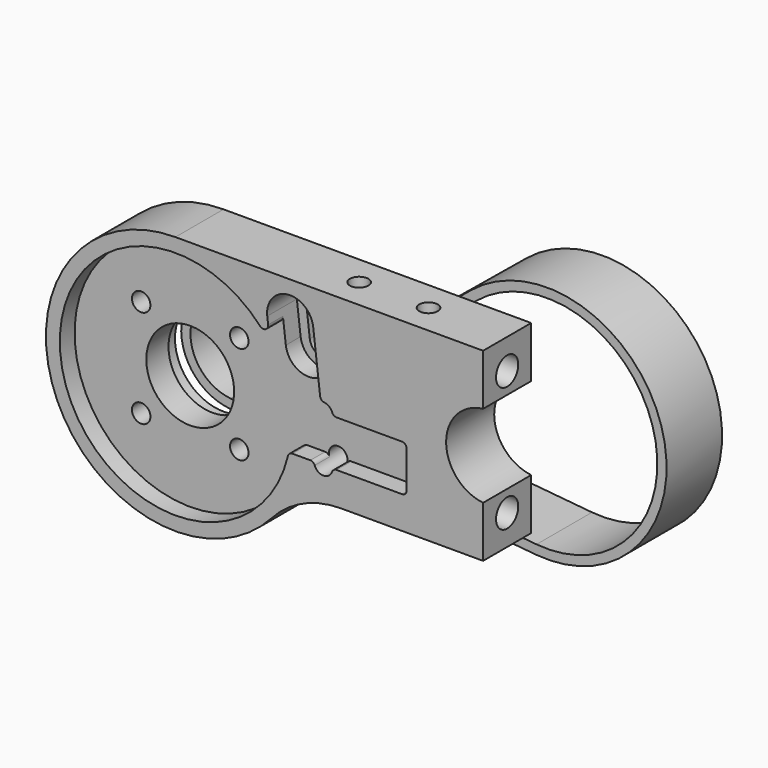
from build123d import *

# Parameters (mm, degrees)
F0_R         = 2
F0_R_2       = 9
F1_DEPTH     = 9
F2_R         = 9.5
F3_DEPTH     = 9
F4_R         = 25
F5_DEPTH     = 4
F8_DEPTH     = 8
F10_DEPTH    = 5.001
F11_R        = 1
F13_DEPTH    = 4
F14_R        = 1
F16_R        = 2
F17_DEPTH    = 13.001
F18_T1_DEPTH = 6.0710678119
F18_T3_DEPTH = 6.4150512427
F20_DEPTH    = 3
F21_R        = 3
F22_DEPTH    = 14
F25_DEPTH    = 15
F26_R        = 2
F27_DEPTH    = 14
F28_R        = 3.75
F29_DEPTH    = 3.5
F30_R        = 10.5
F31_DEPTH    = 3


# Not quite as in the source:
# - a fillet or chamfer that OpenCascade refuses, or shapes differently, is made with other operations: its cross-section is extruded or revolved along the edge and cut away or added


with BuildPart() as f1:
    # F0 (on Front) → F1 (new body)
    with BuildSketch(Plane.XZ):
        with BuildLine():
            ThreePointArc((66.5277720645, -0.94427191), (58.5277720645, 8), (66.5277720645, 16.94427191))
            Line((66.5277720645, 16.94427191), (66.5277720645, 28))
            Line((66.5277720645, 28), (0, 28))
            ThreePointArc((0, 28), (-25.5603860169, -11.430952133), (20.86996779, -18.6666666667))
            ThreePointArc((20.86996779, -18.6666666667), (27.6121218307, -13.7425814165), (35.77708764, -12))
            Line((35.77708764, -12), (66.5277720645, -12))
            Line((66.5277720645, -12), (66.5277720645, -0.94427191))
        make_face()
        with Locations((-10.6066017178, -10.6066017178)):
            Circle(F0_R, mode=Mode.SUBTRACT)
        with Locations((10.6066017178, -10.6066017178)):
            Circle(F0_R, mode=Mode.SUBTRACT)
        with Locations((-10.6066017178, 10.6066017178)):
            Circle(F0_R, mode=Mode.SUBTRACT)
        Circle(F0_R_2, mode=Mode.SUBTRACT)
        with Locations((10.6066017178, 10.6066017178)):
            Circle(F0_R, mode=Mode.SUBTRACT)
    extrude(amount=F1_DEPTH)

    # F2 (on face) → F3 (cut)
    with BuildSketch(Plane(origin=(0, 0, 0), x_dir=(-1, 0, 0), z_dir=(0, 1, 0))):
        Circle(F2_R)
    extrude(amount=-F3_DEPTH, mode=Mode.SUBTRACT)

    # F4 (on face) → F5 (join)
    with BuildSketch(Plane.XZ.offset(9)):
        with BuildLine():
            Line((66.5277720645, 28), (0, 28))
            ThreePointArc((0, 28), (-25.5603860169, -11.430952133), (20.86996779, -18.6666666667))
            ThreePointArc((20.86996779, -18.6666666667), (27.6121218307, -13.7425814165), (35.77708764, -12))
            Line((35.77708764, -12), (66.5277720645, -12))
            Line((66.5277720645, -12), (66.5277720645, -0.94427191))
            ThreePointArc((66.5277720645, -0.94427191), (58.5277720645, 8), (66.5277720645, 16.94427191))
            Line((66.5277720645, 16.94427191), (66.5277720645, 28))
        make_face()
        Circle(F4_R, mode=Mode.SUBTRACT)
    extrude(amount=F5_DEPTH)

    # F7 (on face) → F8 (cut)
    with BuildSketch(Plane.XZ.offset(13)):
        with BuildLine():
            ThreePointArc((20.6707497856, 12.5187900095), (26.2242624374, 8.1417479459), (30.601304501, 13.6952605977))
            Line((30.601304501, 13.6952605977), (29.7846953358, 20.5882352941))
            ThreePointArc((29.7846953358, 20.5882352941), (24.231182684, 24.9652773577), (19.8541406204, 19.4117647059))
            Line((19.8541406204, 19.4117647059), (20.6707497856, 12.5187900095))
        make_face()
    extrude(amount=-F8_DEPTH, mode=Mode.SUBTRACT)

    # F9 (on face) → F10 (cut, through all)
    with BuildSketch(Plane.XZ.offset(5)):
        with BuildLine():
            ThreePointArc((27.7985843927, 20.3529411765), (24.4664768016, 22.9791664146), (21.8402515635, 19.6470588235))
            Line((21.8402515635, 19.6470588235), (22.6568607287, 12.7540841271))
            ThreePointArc((22.6568607287, 12.7540841271), (25.9889683197, 10.127858889), (28.6151935579, 13.4599664801))
            Line((28.6151935579, 13.4599664801), (27.7985843927, 20.3529411765))
        make_face()
    extrude(amount=-F10_DEPTH, mode=Mode.SUBTRACT)

    # F11
    f11_edges = [f1.edges().sort_by_distance(p)[0] for p in [
        (20.450239, -11, 14.380116),
        (23.474902, -11, 8.598196),
    ]]
    fillet(f11_edges, radius=F11_R)

    # F12 (on face) → F13 (cut, through all)
    with BuildSketch(Plane.XZ.offset(13)):
        with BuildLine():
            ThreePointArc((24.038630661, 6.8661660296), (24.9815394091, 0.9605668915), (24.4948974278, -5))
            Line((24.4948974278, -5), (50, -5))
            Line((50, -5), (50, 0))
            Line((50, 0), (50, 5))
            Line((50, 5), (31.6314300723, 5))
            Line((31.6314300723, 5), (30.601304501, 13.6952605977))
            ThreePointArc((30.601304501, 13.6952605977), (29.192263391, 9.5923156783), (25.1061510967, 8.1351814429))
            ThreePointArc((25.1061510967, 8.1351814429), (24.2349308003, 7.7845517146), (24.038630661, 6.8661660296))
        make_face()
    extrude(amount=-F13_DEPTH, mode=Mode.SUBTRACT)

    # F14
    f14_edges = [f1.edges().sort_by_distance(p)[0] for p in [
        (24.494897, -11, -5),
        (50, -11, 5),
        (50, -11, -5),
    ]]
    fillet(f14_edges, radius=F14_R)

    # F16 (on face) → F17 (cut, through all)
    with BuildSketch(Plane.XZ.offset(13)):
        with Locations((32, 5)):
            Circle(F16_R)
        with Locations((32, -5)):
            Circle(F16_R)
    extrude(amount=-F17_DEPTH, mode=Mode.SUBTRACT)

    # F18: fillet of radius 1 on 4 edges, made by hand

    # F18_s2 → F18_t1 (cut)
    with BuildSketch(Plane.XZ.offset(9)):
        with BuildLine():
            ThreePointArc((34.8284271248, -5), (34.2510768556, -5.1835034191), (33.8856180832, -5.6666666667))
            ThreePointArc((33.8856180832, -5.6666666667), (33.9711971193, -5.3382039575), (34, -5))
            Line((34, -5), (34.8284271248, -5))
        make_face()
        with BuildLine():
            ThreePointArc((29.1715728752, -5), (29.7489231444, -5.1835034191), (30.1143819168, -5.6666666667))
            ThreePointArc((30.1143819168, -5.6666666667), (30.0288028807, -5.3382039575), (30, -5))
            Line((30, -5), (29.1715728752, -5))
        make_face()
        with BuildLine():
            ThreePointArc((34.8284271248, 5), (34.2510768556, 5.1835034191), (33.8856180832, 5.6666666667))
            ThreePointArc((33.8856180832, 5.6666666667), (33.9711971193, 5.3382039575), (34, 5))
            Line((34, 5), (34.8284271248, 5))
        make_face()
    extrude(amount=F18_T1_DEPTH, mode=Mode.SUBTRACT)

    # F18_s4 → F18_t3 (cut)
    with BuildSketch(Plane.XZ.offset(9)):
        with BuildLine():
            ThreePointArc((32.1897446196, 6.9909788998), (31.5856544625, 7.2713099967), (31.2915614579, 7.8688212908))
            Line((31.2915614579, 7.8688212908), (31.4052109282, 6.9095093506))
            ThreePointArc((31.4052109282, 6.9095093506), (31.7934217487, 6.9893027487), (32.1897446196, 6.9909788998))
        make_face()
    extrude(amount=F18_T3_DEPTH, mode=Mode.SUBTRACT)

    # F19 (on face) → F20 (cut)
    with BuildSketch(Plane(origin=(0, 0, 0), x_dir=(-1, 0, 0), z_dir=(0, 1, 0))):
        with BuildLine():
            ThreePointArc((-30, 5), (-32, 7), (-34, 5))
            Line((-34, 5), (-34, -5))
            ThreePointArc((-34, -5), (-32, -7), (-30, -5))
            Line((-30, -5), (-30, 5))
        make_face()
    extrude(amount=-F20_DEPTH, mode=Mode.SUBTRACT)

    # F21 (on face) → F22 (cut)
    with BuildSketch(Plane.YZ.offset(66.5277720645)):
        with Locations((-6.5, 21.5)):
            Circle(F21_R)
        with Locations((-6.5, -5.5)):
            Circle(F21_R)
    extrude(amount=-F22_DEPTH, mode=Mode.SUBTRACT)

    # F26 (on face) → F27 (cut)
    with BuildSketch(Plane.XY.offset(28)):
        with Locations((49.5277720645, -6.5)):
            Circle(F26_R)
        with Locations((34.5277720645, -6.5)):
            Circle(F26_R)
    extrude(amount=-F27_DEPTH, mode=Mode.SUBTRACT)

    # F28 (on face) → F29 (cut)
    with BuildSketch(Plane(origin=(0, 0, 0), x_dir=(-1, 0, 0), z_dir=(0, 1, 0))):
        with Locations((-10.6066017178, -10.6066017178)):
            Circle(F28_R)
        with Locations((10.6066017178, -10.6066017178)):
            Circle(F28_R)
        with Locations((10.6066017178, 10.6066017178)):
            Circle(F28_R)
        with Locations((-10.6066017178, 10.6066017178)):
            Circle(F28_R)
    extrude(amount=-F29_DEPTH, mode=Mode.SUBTRACT)

    # F30 (on face) → F31 (cut)
    with BuildSketch(Plane(origin=(0, 0, 0), x_dir=(-1, 0, 0), z_dir=(0, 1, 0))):
        Circle(F30_R)
    extrude(amount=-F31_DEPTH, mode=Mode.SUBTRACT)


with BuildPart() as f25:
    # F24 (on offset) → F25 (new body)
    with BuildSketch(Plane(origin=(0, 3, 0), x_dir=(-1, 0, 0), z_dir=(0, 1, 0))):
        with BuildLine():
            Line((-30.2365222754, 10.8918314545), (-51.1259867982, 28.0124227688))
            ThreePointArc((-51.1259867982, 28.0124227688), (-92.2766057305, 15.5505534348), (-65.0905572844, -17.759961357))
            Line((-65.0905572844, -17.759961357), (1.0879161627, -11.4986494173))
            ThreePointArc((1.0879161627, -11.4986494173), (11.4944642154, 1.1312790991), (-1.1746259412, 11.4901154867))
            Line((-1.1746259412, 11.4901154867), (-24.3518451825, 9.1207256405))
            ThreePointArc((-24.3518451825, 9.1207256405), (-27.471031774, 9.4186831416), (-30.2365222754, 10.8918314545))
        make_face()
        with BuildLine():
            ThreePointArc((-65.2789410355, -15.7688532328), (-90.3636524037, 14.966935778), (-52.39375764, 26.4655688349))
            Line((-52.39375764, 26.4655688349), (-31.5042931172, 9.3449775207))
            ThreePointArc((-31.5042931172, 9.3449775207), (-28.0474299905, 7.5035421295), (-24.1484467511, 7.1310952532))
            Line((-24.1484467511, 7.1310952532), (-0.9712275098, 9.5004850994))
            ThreePointArc((-0.9712275098, 9.5004850994), (9.5040808015, 0.9353866144), (0.8995324116, -9.5075412931))
            Line((0.8995324116, -9.5075412931), (-65.2789410355, -15.7688532328))
        make_face(mode=Mode.SUBTRACT)
    extrude(amount=F25_DEPTH)


solid = Compound([f1.part, f25.part])
